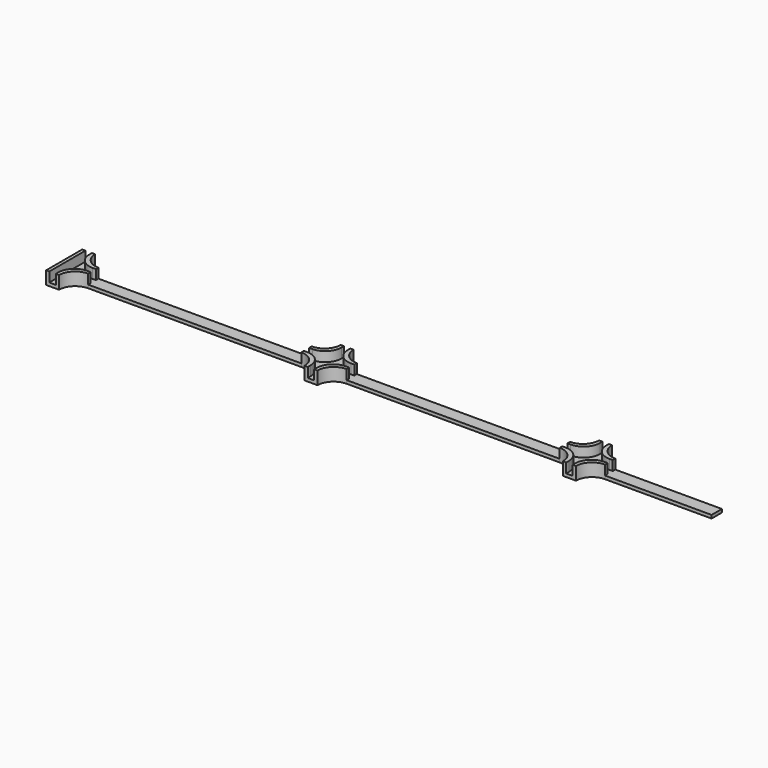
from build123d import *

# Parameters (mm, degrees)
F0_W     = 4
F0_H     = 4
F0_H_2   = 5
F0_W_2   = 76
F0_H_3   = 2.5597222634
F0_H_4   = 2.4402777366
F0_W_3   = 38
F1_DEPTH = 1
F2_W     = 1
F2_H     = 14
F2_H_2   = 5
F3_DEPTH = 3
F4_R     = 4.99999
F2_W_2   = 5
F2_H_3   = 1
F5_DEPTH = 3
F6_R     = 4.99999
F7_DEPTH = 3
F8_R     = 4.99999


# Not quite as in the source:
# - a fillet or chamfer is up to 0.001 mm smaller than in the source, because OpenCascade refuses the exact size


with BuildPart() as f1:
    # F0 (on Top) → F1 (new body)
    with BuildSketch(Plane.XY):
        Polygon((-101, 2), (-97, 2), (-97, 4.5597222634), (-97, 7), (-101, 7), align=None)
        with Locations((-99, 0)):
            Rectangle(F0_W, F0_H)
        with Locations((-99, -4.5)):
            Rectangle(F0_W, F0_H_2)
        with Locations((-59, 0)):
            Rectangle(F0_W_2, F0_H)
        with Locations((-19, 3.2798611317)):
            Rectangle(F0_W, F0_H_3)
        with Locations((-19, 0)):
            Rectangle(F0_W, F0_H)
        with Locations((-19, -4.5)):
            Rectangle(F0_W, F0_H_2)
        with Locations((-19, 5.7798611317)):
            Rectangle(F0_W, F0_H_4)
        with Locations((21, 0)):
            Rectangle(F0_W_2, F0_H)
        with Locations((61, 5.7798611317)):
            Rectangle(F0_W, F0_H_4)
        with Locations((61, 3.2798611317)):
            Rectangle(F0_W, F0_H_3)
        with Locations((61, -4.5)):
            Rectangle(F0_W, F0_H_2)
        with Locations((61, 0)):
            Rectangle(F0_W, F0_H)
        with Locations((82, 0)):
            Rectangle(F0_W_3, F0_H)
    extrude(amount=F1_DEPTH)

    # F2 (on face) → F3 (join)
    with BuildSketch(Plane.XY.offset(1)):
        with Locations((-100.5, 0)):
            Rectangle(F2_W, F2_H)
        with Locations((-97.5, 4.5)):
            Rectangle(F2_W, F2_H_2)
        Polygon((-97, 2), (-98, 2), (-98, 1), (-92, 1), (-92, 2), align=None)
        Polygon((-98, -1), (-98, -2), (-97, -2), (-92, -2), (-92, -1), align=None)
        with Locations((-97.5, -4.5)):
            Rectangle(F2_W, F2_H_2)
    extrude(amount=F3_DEPTH)

    # F4 (radius 5 in the source; OpenCascade refuses exactly that, so slightly less here)
    f4_edges = [f1.edges().sort_by_distance(p)[0] for p in [
        (-97, -2, 2),
        (-98, 1, 2.5),
        (-98, -1, 2.5),
        (-97, 2, 2),
    ]]
    fillet(f4_edges, radius=F4_R)

    # F2 (on face) → F5 (join)
    with BuildSketch(Plane.XY.offset(1)):
        Polygon((-21, 7), (-21, 2), (-21, 1), (-20, 1), (-20, 7), align=None)
        Polygon((-17, 7), (-18, 7), (-18, 1), (-17, 1), (-17, 2), align=None)
        with Locations((-14.5, 1.5)):
            Rectangle(F2_W_2, F2_H_3)
        with Locations((-23.5, 1.5)):
            Rectangle(F2_W_2, F2_H_3)
        with Locations((-23.5, -1.5)):
            Rectangle(F2_W_2, F2_H_3)
        Polygon((-21, -1), (-21, -2), (-21, -7), (-20, -7), (-20, -1), align=None)
        with Locations((-14.5, -1.5)):
            Rectangle(F2_W_2, F2_H_3)
        Polygon((-18, -1), (-18, -7), (-17, -7), (-17, -2), (-17, -1), align=None)
    extrude(amount=F5_DEPTH)

    # F6 (radius 5 in the source; OpenCascade refuses exactly that, so slightly less here)
    f6_edges = [f1.edges().sort_by_distance(p)[0] for p in [
        (-18, 1, 2.5),
        (-20, 1, 2.5),
        (-17, -2, 2),
        (-20, -1, 2.5),
        (-21, -2, 2),
        (-21, 2, 2),
        (-17, 2, 2),
        (-18, -1, 2.5),
    ]]
    fillet(f6_edges, radius=F6_R)

    # F2 (on face) → F7 (join)
    with BuildSketch(Plane.XY.offset(1)):
        Polygon((59, 7), (59, 2), (59, 1), (60, 1), (60, 7), align=None)
        with Locations((65.5, 1.5)):
            Rectangle(F2_W_2, F2_H_3)
        Polygon((63, 7), (62, 7), (62, 1), (63, 1), (63, 2), align=None)
        with Locations((65.5, -1.5)):
            Rectangle(F2_W_2, F2_H_3)
        Polygon((62, -1), (62, -7), (63, -7), (63, -2), (63, -1), align=None)
        with Locations((56.5, 1.5)):
            Rectangle(F2_W_2, F2_H_3)
        with Locations((56.5, -1.5)):
            Rectangle(F2_W_2, F2_H_3)
        Polygon((59, -1), (59, -2), (59, -7), (60, -7), (60, -1), align=None)
    extrude(amount=F7_DEPTH)

    # F8 (radius 5 in the source; OpenCascade refuses exactly that, so slightly less here)
    f8_edges = [f1.edges().sort_by_distance(p)[0] for p in [
        (63, -2, 2),
        (60, 1, 2.5),
        (62, 1, 2.5),
        (60, -1, 2.5),
        (62, -1, 2.5),
        (59, -2, 2),
        (59, 2, 2),
        (63, 2, 2),
    ]]
    fillet(f8_edges, radius=F8_R)


solid = f1.part
